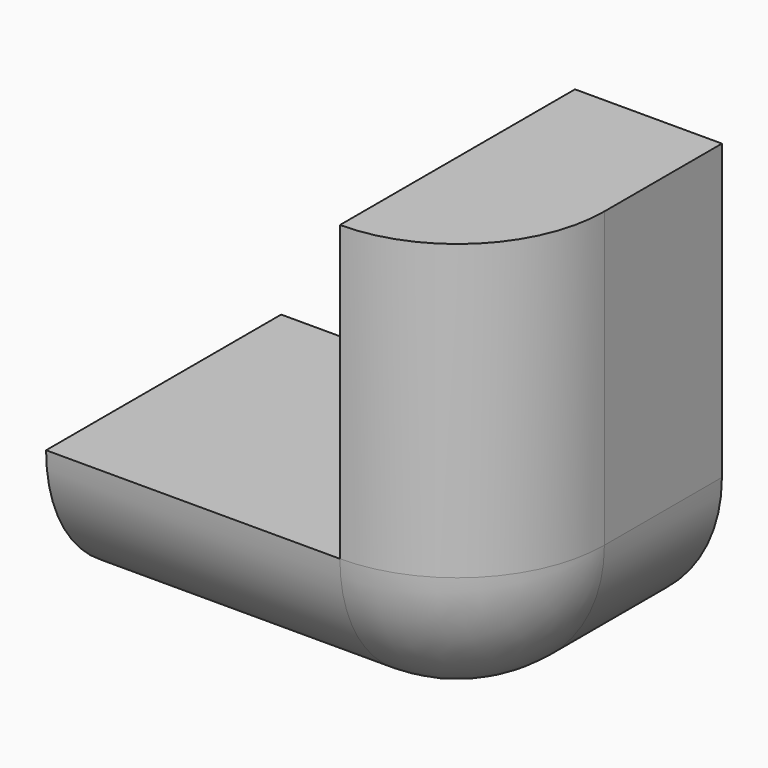
from build123d import *

# Parameters (mm, degrees)
F0_W     = 228.6
F0_H     = 76.2
F1_DEPTH = 152.4
F2_W     = 152.4
F2_H     = 152.4
F2_H_2   = 76.2
F3_DEPTH = 76.2
F4_R     = 76.2
F5_R     = 76.19999


# Not quite as in the source:
# - a fillet or chamfer is up to 0.001 mm smaller than in the source, because OpenCascade refuses the exact size


with BuildPart() as f1:
    # F0 (on Front) → F1 (new body)
    with BuildSketch(Plane.XZ):
        with Locations((-3.7755966187, 13.4019921658)):
            Rectangle(F0_W, F0_H)
    extrude(amount=F1_DEPTH)

    # F2 (on face) → F3 (join)
    with BuildSketch(Plane.YZ.offset(110.5244033813)):
        with Locations((-76.2, 127.7019921658)):
            Rectangle(F2_W, F2_H)
        with Locations((-76.2, 13.4019921658)):
            Rectangle(F2_W, F2_H_2)
    extrude(amount=-F3_DEPTH)

    # F4
    f4_edges = [f1.edges().sort_by_distance(p)[0] for p in [
        (-3.775597, -152.4, -24.698008),
    ]]
    fillet(f4_edges, radius=F4_R)

    # F5 (radius 76.2 in the source; OpenCascade refuses exactly that, so slightly less here)
    f5_edges = [f1.edges().sort_by_distance(p)[0] for p in [
        (110.524403, -152.4, 127.701992),
    ]]
    fillet(f5_edges, radius=F5_R)


solid = f1.part
